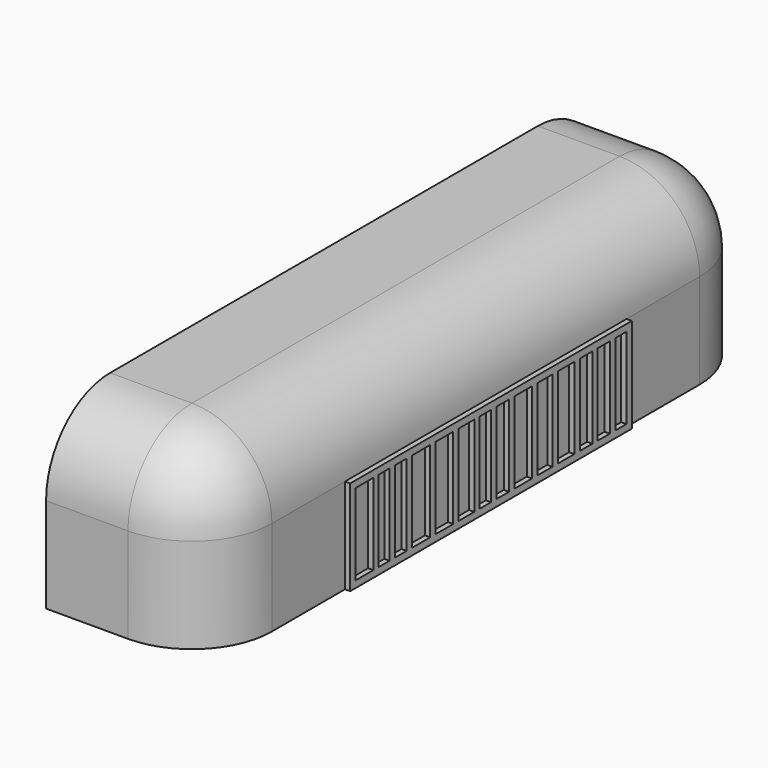
from build123d import *

# Parameters (mm, degrees)
F0_W     = 44.1192735617
F0_H     = 11.1166509635
F1_DEPTH = 5.14096
F2_R     = 5.08
F3_R     = 5.08
F4_W     = 1.4028784636
F4_H     = 5.165201461
F4_W_2   = 0.8638333529
F4_W_3   = 0.9213921431
F4_W_4   = 1.4403553497
F4_W_5   = 1.3910879198
F4_W_6   = 1.2432860676
F4_W_7   = 0.8935106736
F4_W_8   = 1.0018550383
F4_W_9   = 1.3910882691
F4_W_10  = 1.1940188706
F4_W_11  = 1.3041589975
F4_W_12  = 0.9969494123
F4_W_13  = 0.9587099776
F4_W_14  = 0.8777634058
F5_DEPTH = 0.3302


# Not quite as in the source:
# - a feature names something its author has since deleted; it is built from what else it names


with BuildPart() as f1:
    # F0 (on Right) → F1 (new body, symmetric)
    with BuildSketch(Plane.YZ):
        Rectangle(F0_W, F0_H)
    extrude(amount=F1_DEPTH, both=True)

    # F2
    f2_edges = [f1.edges().sort_by_distance(p)[0] for p in [
        (5.14096, 22.059637, 0),
        (5.14096, -22.059637, 0),
    ]]
    fillet(f2_edges, radius=F2_R)

    # F3
    f3_edges = [f1.edges().sort_by_distance(p)[0] for p in [
        (-2.54, 22.059637, 5.558325),
    ]]
    fillet(f3_edges, radius=F3_R)

    # F4 (on face) → F5 (join)
    with BuildSketch(Plane.YZ.offset(5.14096)):
        Polygon((9.4375805929, -5.5583254817), (11.1789442599, -5.5583254817), (11.1789442599, 0.4704763523), (8.4788706154, 0.4704763523), (7.0501212031, 0.4704763523), (4.8823622055, 0.4704763523), (3.2565433066, 0.4704763523), (1.4336550375, 0.4704763523), (0, 0.4704763523), (-1.3253106736, 0.4704763523), (-3.0003967695, 0.4704763523), (-4.8232846893, 0.4704763523), (-6.695440039, 0.4704763523), (-11.1789442599, 0.4704763523), (-11.1789442599, -5.5583254817), (-8.9124655351, -5.5583254817), (-6.695440039, -5.5583254817), (-4.8232846893, -5.5583254817), (-3.0003967695, -5.5583254817), (-1.3253106736, -5.5583254817), (0, -5.5583254817), (1.4336550375, -5.5583254817), (3.2565433066, -5.5583254817), (4.8823622055, -5.5583254817), (7.0501212031, -5.5583254817), (8.4788706154, -5.5583254817), align=None)
        with Locations((-10.0457047669, -2.5439243782)):
            Rectangle(F4_W, F4_H, mode=Mode.SUBTRACT)
        with Locations((-8.4805488586, -2.5439243782)):
            Rectangle(F4_W_2, F4_H, mode=Mode.SUBTRACT)
        with Locations((-7.1561361106, -2.5439243782)):
            Rectangle(F4_W_3, F4_H, mode=Mode.SUBTRACT)
        with Locations((-5.5434623642, -2.5439243782)):
            Rectangle(F4_W_4, F4_H, mode=Mode.SUBTRACT)
        with Locations((-3.6959407294, -2.5439243782)):
            Rectangle(F4_W_5, F4_H, mode=Mode.SUBTRACT)
        with Locations((-1.9469537074, -2.5439243782)):
            Rectangle(F4_W_6, F4_H, mode=Mode.SUBTRACT)
        with Locations((-0.4467553368, -2.5439243782)):
            Rectangle(F4_W_7, F4_H, mode=Mode.SUBTRACT)
        with Locations((0.9327275184, -2.5439243782)):
            Rectangle(F4_W_8, F4_H, mode=Mode.SUBTRACT)
        with Locations((2.5609991721, -2.5439243782)):
            Rectangle(F4_W_9, F4_H, mode=Mode.SUBTRACT)
        with Locations((4.2853527702, -2.5439243782)):
            Rectangle(F4_W_10, F4_H, mode=Mode.SUBTRACT)
        with Locations((5.9662417043, -2.5439243782)):
            Rectangle(F4_W_11, F4_H, mode=Mode.SUBTRACT)
        with Locations((7.5485959092, -2.5439243782)):
            Rectangle(F4_W_12, F4_H, mode=Mode.SUBTRACT)
        with Locations((8.9582256041, -2.5439243782)):
            Rectangle(F4_W_13, F4_H, mode=Mode.SUBTRACT)
        with Locations((10.3082622958, -2.5439243782)):
            Rectangle(F4_W_14, F4_H, mode=Mode.SUBTRACT)
    extrude(amount=F5_DEPTH)


solid = f1.part
